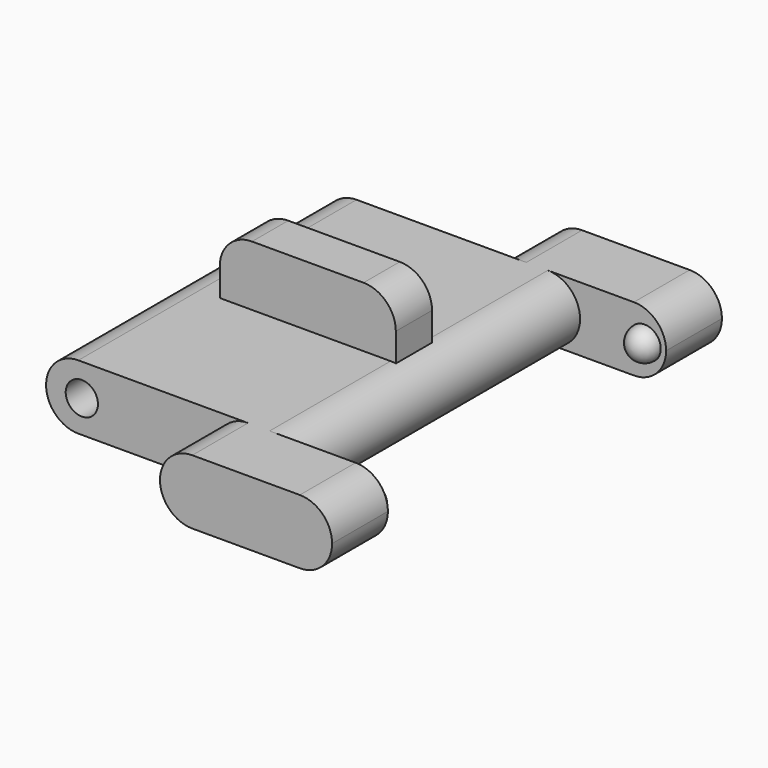
from build123d import *

# Parameters (mm, degrees)
F1_DEPTH      = 3
F2_R          = 0.75
F3_DEPTH      = 0.75
F4_R          = 0.75
F5_DEPTH      = 0.75
F6_R          = 0.75
F7_DEPTH      = 25
F8_R          = 1.49999
F9_W          = 8.1852182662
F9_H          = 2.1034856807
F10_DEPTH     = 2.8
F11_R         = 1.5
F13_DEPTH     = 0.5
F14_R         = 0.74999
F15_T1_DEPTH  = 16.1687540342
F15_T6_DEPTH  = 19.9187540342
F15_T11_DEPTH = 19.9187540342
F15_T17_DEPTH = 19.9187540342
F16_R         = 1.49999


# Not quite as in the source:
# - a fillet or chamfer that OpenCascade refuses, or shapes differently, is made with other operations: its cross-section is extruded or revolved along the edge and cut away or added
# - a fillet or chamfer is up to 0.001 mm smaller than in the source, because OpenCascade refuses the exact size
# - a feature names something its author has since deleted; it is built from what else it names


with BuildPart() as f1:
    # F0 (on Top) → F1 (new body)
    with BuildSketch(Plane.XY):
        Polygon((0, 16.1687540342), (0, 0), (7.8920411056, 0), (11.8920411056, 0), (11.8920411056, 16.1687540342), (7.8920411056, 16.1687540342), align=None)
        Polygon((7.8920411056, 19.412382182), (7.8920411056, 16.1687540342), (11.8920411056, 16.1687540342), (15.8920411056, 16.1687540342), (15.8920411056, 19.412382182), align=None)
        Polygon((11.8920411056, 0), (7.8920411056, 0), (7.8920411056, -3.2436281478), (15.8920411056, -3.2436281478), (15.8920411056, 0), align=None)
    extrude(amount=F1_DEPTH)

    # F2 (on face) → F3 (join)
    with BuildSketch(Plane.XZ.offset(-16.1687540342)):
        with Locations((14.8920411056, 1.5)):
            Circle(F2_R)
    extrude(amount=F3_DEPTH)

    # F4 (on face) → F5 (join)
    with BuildSketch(Plane(origin=(0, 0, 0), x_dir=(-1, 0, 0), z_dir=(0, 1, 0))):
        with Locations((-14.8920411056, 1.5)):
            Circle(F4_R)
    extrude(amount=F5_DEPTH)

    # F6 (on face) → F7 (cut)
    with BuildSketch(Plane.XZ):
        with Locations((1.6622071853, 1.5)):
            Circle(F6_R)
    extrude(amount=-F7_DEPTH, mode=Mode.SUBTRACT)

    # F8 (radius 1.5 in the source; OpenCascade refuses exactly that, so slightly less here)
    f8_edges = [f1.edges().sort_by_distance(p)[0] for p in [
        (0, 8.084377, 3),
        (0, 8.084377, 0),
        (15.892041, 17.790568, 3),
        (15.892041, 17.790568, 0),
        (15.892041, -1.621814, 3),
        (15.892041, -1.621814, 0),
    ]]
    fillet(f8_edges, radius=F8_R)

    # F9 (on face) → F10 (join)
    with BuildSketch(Plane.XY.offset(3)):
        with Locations((6.5418113065, 8.0843770171)):
            Rectangle(F9_W, F9_H)
    extrude(amount=F10_DEPTH)

    # F11
    f11_edges = [f1.edges().sort_by_distance(p)[0] for p in [
        (10.63442, 8.084377, 5.8),
        (2.449202, 8.084377, 5.8),
    ]]
    fillet(f11_edges, radius=F11_R)

    # F12 (on face) → F13 (cut)
    with BuildSketch(Plane(origin=(0, 0, 0), x_dir=(1, 0, 0), z_dir=(0, 0, -1))):
        Polygon((5.4570450447, -1.8034656052), (2.8651286848, -8.0843770171), (5.4570450447, -14.365288429), (6.276931148, -14.365288429), (3.6494208034, -8.0843770171), (6.276931148, -1.8034656052), align=None)
        Polygon((7.7570450447, -1.8034656052), (5.1651286848, -8.0843770171), (7.7570450447, -14.365288429), (8.576931148, -14.365288429), (5.9494208034, -8.0843770171), (8.576931148, -1.8034656052), align=None)
    extrude(amount=-F13_DEPTH, mode=Mode.SUBTRACT)

    # F14 (radius 0.75 in the source; OpenCascade refuses exactly that, so slightly less here)
    f14_edges = [f1.edges().sort_by_distance(p)[0] for p in [
        (15.642041, 0.75, 1.5),
        (14.142041, 15.418754, 1.5),
    ]]
    fillet(f14_edges, radius=F14_R)

    # F15: fillet of radius 1.5 on 2 edges, made by hand

    # F15_s2 → F15_t1 (cut)
    with BuildSketch(Plane.XZ.offset(-16.1687540342)):
        with BuildLine():
            ThreePointArc((10.3920411056, 0), (11.4527012774, 0.4393398282), (11.8920411056, 1.5))
            Line((11.8920411056, 1.5), (11.8920411056, 0))
            Line((11.8920411056, 0), (10.3920411056, 0))
        make_face()
    extrude(amount=F15_T1_DEPTH, mode=Mode.SUBTRACT)


with BuildPart() as f15_tool4:
    # F15_s5 → F15_t6 (new body)
    with BuildSketch(Plane.XZ):
        with BuildLine():
            ThreePointArc((10.3920411056, 3), (11.4527012774, 2.5606601718), (11.8920411056, 1.5))
            Line((11.8920411056, 1.5), (11.8920411056, 3))
            Line((11.8920411056, 3), (10.3920411056, 3))
        make_face()
    extrude(amount=-F15_T6_DEPTH)

    split(bisect_by=Plane.XZ.offset(-7.0326341767), keep=Keep.TOP)


with BuildPart() as f1_1:
    add(f1.part)

    # F15_t3: cut F15_tool4
    add(f15_tool4.part, mode=Mode.SUBTRACT)


with BuildPart() as f15_tool9:
    # F15_s10 → F15_t11 (new body)
    with BuildSketch(Plane.XZ.offset(3.75)):
        with BuildLine():
            ThreePointArc((10.3920411056, 3), (11.4527012774, 2.5606601718), (11.8920411056, 1.5))
            Line((11.8920411056, 1.5), (11.8920411056, 3))
            Line((11.8920411056, 3), (10.3920411056, 3))
        make_face()
    extrude(amount=-F15_T11_DEPTH)

    split(bisect_by=Plane.XZ.offset(-7.0326341767), keep=Keep.BOTTOM)

    split(bisect_by=Plane.YZ.offset(10.6344204396), keep=Keep.TOP)


with BuildPart() as f1_2:
    add(f1_1.part)

    # F15_t8: cut F15_tool9
    add(f15_tool9.part, mode=Mode.SUBTRACT)


with BuildPart() as f15_tool15:
    # F15_s16 → F15_t17 (new body)
    with BuildSketch(Plane.XZ.offset(3.75)):
        with BuildLine():
            ThreePointArc((10.3920411056, 3), (11.4527012774, 2.5606601718), (11.8920411056, 1.5))
            Line((11.8920411056, 1.5), (11.8920411056, 3))
            Line((11.8920411056, 3), (10.3920411056, 3))
        make_face()
    extrude(amount=-F15_T17_DEPTH)

    split(bisect_by=Plane.XZ.offset(-9.1361198574), keep=Keep.BOTTOM)


with BuildPart() as f1_3:
    add(f1_2.part)

    # F15_t14: cut F15_tool15
    add(f15_tool15.part, mode=Mode.SUBTRACT)

    # F16 (radius 1.5 in the source; OpenCascade refuses exactly that, so slightly less here)
    f16_edges = [f1_3.edges().sort_by_distance(p)[0] for p in [
        (7.892041, -1.621814, 3),
        (7.892041, -1.621814, 0),
        (7.892041, 17.790568, 3),
        (7.892041, 17.790568, 0),
    ]]
    fillet(f16_edges, radius=F16_R)


solid = f1_3.part
